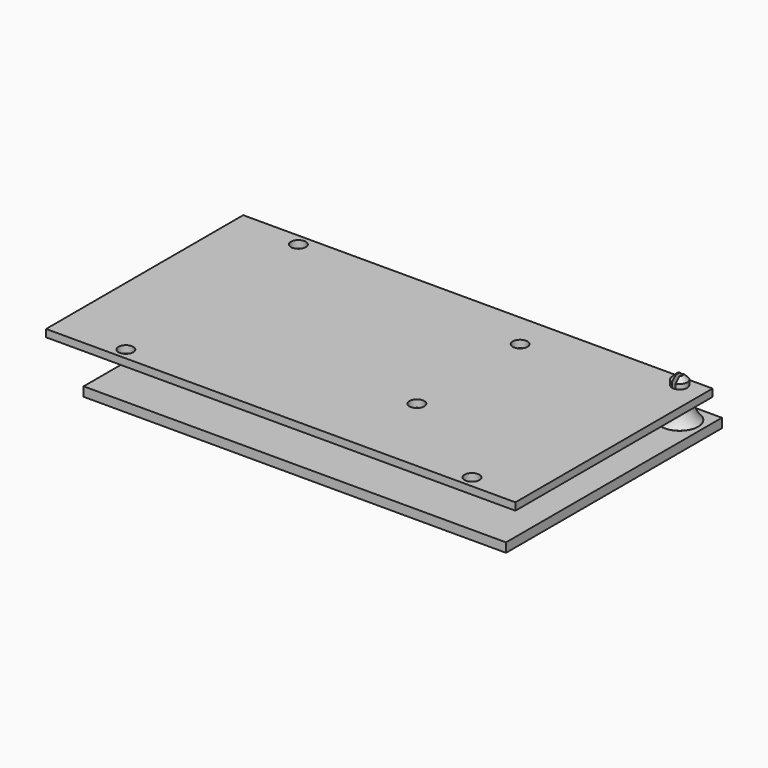
from build123d import *

# Parameters (mm, degrees)
F0_W      = 101.6
F0_H      = 53.340000001
F0_R      = 1.6
F1_DEPTH  = 1.6
F2_R      = 2.540005794
F3_DEPTH  = 5
F4_R      = 1.5
F5_DEPTH  = 3.7
F6_R      = 1.65
F6_R_2    = 1.5
F7_DEPTH  = 2
F8_SIZE   = 1
F10_DEPTH = 3.7
F11_W     = 91.44
F11_H     = 58.4199999868
F12_DEPTH = 2
F13_R     = 4
F14_DEPTH = 0.01


# Not quite as in the source:
# - a fillet or chamfer that OpenCascade refuses, or shapes differently, is made with other operations: its cross-section is extruded or revolved along the edge and cut away or added


with BuildPart() as f1:
    # F0 (on Top) → F1 (new body)
    with BuildSketch(Plane.XY):
        Rectangle(F0_W, F0_H)
        with Locations((-35.56, -24.1300057803)):
            Circle(F0_R, mode=Mode.SUBTRACT)
        with Locations((39.37, -24.1300057803)):
            Circle(F0_R, mode=Mode.SUBTRACT)
        with Locations((15.24, -8.8900057929)):
            Circle(F0_R, mode=Mode.SUBTRACT)
        with Locations((-36.83, 24.1299942065)):
            Circle(F0_R, mode=Mode.SUBTRACT)
        with Locations((15.24, 19.0499942107)):
            Circle(F0_R, mode=Mode.SUBTRACT)
        with Locations((45.72, 24.1299942065)):
            Circle(F0_R, mode=Mode.SUBTRACT)
    extrude(amount=F1_DEPTH)


with BuildPart() as f3:
    # F2 (on face) → F3 (new body)
    with BuildSketch(Plane(origin=(0, 0, 0), x_dir=(1, 0, 0), z_dir=(0, 0, -1))):
        with Locations((45.72, -24.1299942065)):
            Circle(F2_R)
    extrude(amount=F3_DEPTH)

    # F4 (on face) → F5 (join)
    with BuildSketch(Plane.XY):
        with Locations((45.72, 24.1299942065)):
            Circle(F4_R)
    extrude(amount=F5_DEPTH)

    # F6 (on face) → F7 (join)
    with BuildSketch(Plane.XY.offset(3.7)):
        with Locations((45.72, 24.1299942065)):
            Circle(F6_R)
        with Locations((45.72, 24.1299942065)):
            Circle(F6_R_2, mode=Mode.SUBTRACT)
    extrude(amount=-F7_DEPTH)

    # F8
    f8_edges = [f3.edges().sort_by_distance(p)[0] for p in [
        (44.07, 24.129994, 3.7),
    ]]
    chamfer(f8_edges, length=F8_SIZE)

    # F9 (on face) → F10 (cut)
    with BuildSketch(Plane.XY.offset(3.7)):
        with BuildLine():
            ThreePointArc((46.12, 24.6423417448), (45.72, 24.7799942065), (45.32, 24.6423417448))
            Line((45.32, 24.6423417448), (45.32, 23.6176466682))
            ThreePointArc((45.32, 23.6176466682), (45.72, 23.4799942065), (46.12, 23.6176466682))
            Line((46.12, 23.6176466682), (46.12, 24.6423417448))
        make_face()
        with BuildLine():
            ThreePointArc((46.12, 23.6176466682), (45.72, 23.4799942065), (45.32, 23.6176466682))
            Line((45.32, 23.6176466682), (45.32, 20.7503768898))
            Line((45.32, 20.7503768898), (46.12, 20.7503768898))
            Line((46.12, 20.7503768898), (46.12, 23.6176466682))
        make_face()
        with BuildLine():
            Line((46.12, 27.5096115231), (45.32, 27.5096115231))
            Line((45.32, 27.5096115231), (45.32, 24.6423417448))
            ThreePointArc((45.32, 24.6423417448), (45.72, 24.7799942065), (46.12, 24.6423417448))
            Line((46.12, 24.6423417448), (46.12, 27.5096115231))
        make_face()
    extrude(amount=-F10_DEPTH, mode=Mode.SUBTRACT)

    # F13 (on face) → F14 (join)
    with BuildSketch(Plane(origin=(0, 0, -5), x_dir=(1, 0, 0), z_dir=(0, 0, -1))):
        with Locations((45.72, -24.1299942065)):
            Circle(F13_R)
    extrude(amount=-F14_DEPTH)

    # F15: fillet of radius 5 on 1 edges, made by hand

    # F15_s1 → F15_t2 (revolve)
    with BuildSketch(Plane.XZ.offset(-24.1299942065)):
        with BuildLine():
            ThreePointArc((48.260005794, -1.4589436456), (48.6393982057, -3.3694371721), (49.72, -4.99))
            Line((49.72, -4.99), (48.260005794, -4.99))
            Line((48.260005794, -4.99), (48.260005794, -1.4589436456))
        make_face()
    revolve(axis=Axis((45.72, 24.1299942065, -4.99), (0, 0, 1)))


with BuildPart() as f12:
    # F11 (on face) → F12 (new body)
    with BuildSketch(Plane(origin=(0, 0, -5), x_dir=(1, 0, 0), z_dir=(0, 0, -1))):
        with Locations((5.08, 5.7869e-06)):
            Rectangle(F11_W, F11_H)
    extrude(amount=F12_DEPTH)


solid = Compound([f1.part, f3.part, f12.part])
